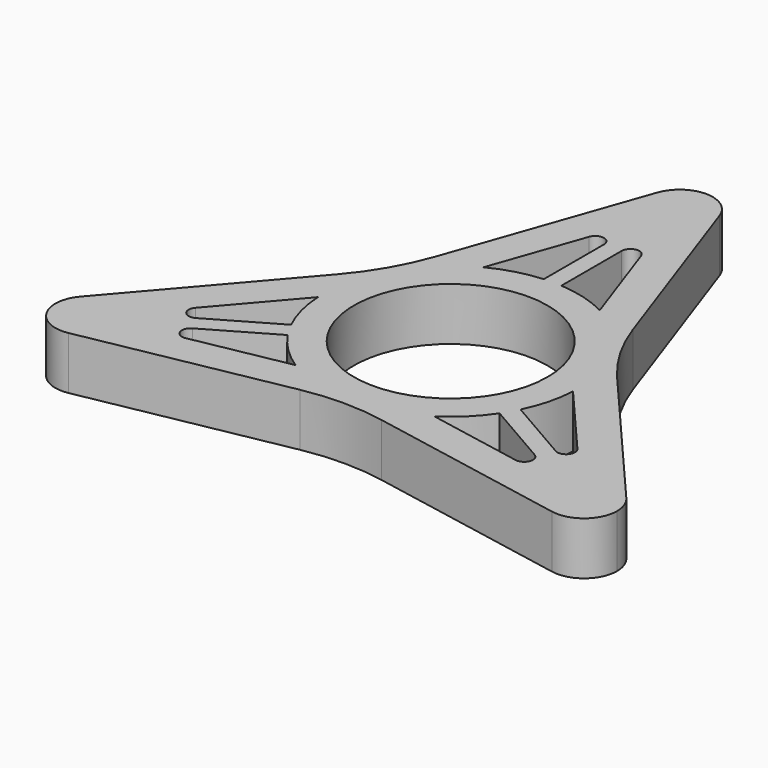
from build123d import *

# Parameters (mm, degrees)
F0_R     = 11
F1_DEPTH = 6


with BuildPart() as f1:
    # F0 (on Top) → F1 (new body)
    with BuildSketch(Plane.XY):
        with BuildLine():
            Line((11.2187429189, 11.8292181419), (3.5389187623, 33.7403846154))
            ThreePointArc((3.5389187623, 33.7403846154), (0, 36.25), (-3.5389187623, 33.7403846154))
            Line((-3.5389187623, 33.7403846154), (-11.2187429189, 11.8292181419))
            ThreePointArc((-11.2187429189, 11.8292181419), (-13.1608995727, 7.5984489111), (-15.8537748772, 3.8011072954))
            Line((-15.8537748772, 3.8011072954), (-30.9894895915, -13.8053987576))
            ThreePointArc((-30.9894895915, -13.8053987576), (-28.3703151015, -12.5067254343), (-25.6147048476, -13.4830653025))
            ThreePointArc((-25.6147048476, -13.4830653025), (-24.8982303588, -14.375), (-24.4840294966, -15.4414524572))
            ThreePointArc((-24.4840294966, -15.4414524572), (-24.4179418082, -15.8433278187), (-24.395825623, -16.25))
            ThreePointArc((-24.395825623, -16.25), (-25.2588111204, -18.643250355), (-27.4505708292, -19.9349858577))
            Line((-27.4505708292, -19.9349858577), (-4.6350319583, -15.6303254372))
            ThreePointArc((-4.6350319583, -15.6303254372), (0, -15.1968978222), (4.6350319583, -15.6303254372))
            Line((4.6350319583, -15.6303254372), (27.4505708292, -19.9349858577))
            ThreePointArc((27.4505708292, -19.9349858577), (25.016299495, -18.3160508741), (24.4840294966, -15.4414524572))
            ThreePointArc((24.4840294966, -15.4414524572), (24.8982303588, -14.375), (25.6147048476, -13.4830653025))
            ThreePointArc((25.6147048476, -13.4830653025), (28.3703151015, -12.5067254343), (30.9894895915, -13.8053987576))
            Line((30.9894895915, -13.8053987576), (15.8537748772, 3.8011072954))
            ThreePointArc((15.8537748772, 3.8011072954), (13.1608995727, 7.5984489111), (11.2187429189, 11.8292181419))
        make_face()
        with BuildLine():
            Line((-19.4313725784, -12.3734087272), (-12.0274698164, -8.0987634745))
            ThreePointArc((-12.0274698164, -8.0987634745), (-10.1599093098, -10.3453488494), (-7.8799155315, -12.171973185))
            Line((-7.8799155315, -12.171973185), (-18.7459713, -14.2220970264))
            ThreePointArc((-18.7459713, -14.2220970264), (-19.8690053401, -13.5870615238), (-19.4313725784, -12.3734087272))
        make_face(mode=Mode.SUBTRACT)
        with BuildLine():
            ThreePointArc((-20.4313725784, -10.6413579197), (-21.7012431124, -10.4135326105), (-21.68968297, -9.1234388512))
            Line((-21.68968297, -9.1234388512), (-14.4811957581, -0.7382204374))
            ThreePointArc((-14.4811957581, -0.7382204374), (-14.0392895695, -3.6260651377), (-13.0274698164, -6.366712667))
            Line((-13.0274698164, -6.366712667), (-20.4313725784, -10.6413579197))
        make_face(mode=Mode.SUBTRACT)
        with BuildLine():
            ThreePointArc((19.4313725784, -12.3734087272), (19.8690053401, -13.5870615238), (18.7459713, -14.2220970264))
            Line((18.7459713, -14.2220970264), (7.8799155315, -12.171973185))
            ThreePointArc((7.8799155315, -12.171973185), (10.1599093098, -10.3453488494), (12.0274698164, -8.0987634745))
            Line((12.0274698164, -8.0987634745), (19.4313725784, -12.3734087272))
        make_face(mode=Mode.SUBTRACT)
        Circle(F0_R, mode=Mode.SUBTRACT)
        with BuildLine():
            Line((14.4811957581, -0.7382204374), (21.68968297, -9.1234388512))
            ThreePointArc((21.68968297, -9.1234388512), (21.7012431124, -10.4135326105), (20.4313725784, -10.6413579197))
            Line((20.4313725784, -10.6413579197), (13.0274698164, -6.366712667))
            ThreePointArc((13.0274698164, -6.366712667), (14.0392895695, -3.6260651377), (14.4811957581, -0.7382204374))
        make_face(mode=Mode.SUBTRACT)
        with BuildLine():
            Line((-6.6012802267, 12.9101936225), (-2.9437116699, 23.3455358777))
            ThreePointArc((-2.9437116699, 23.3455358777), (-1.8322377723, 24.0005941343), (-1, 23.0147666469))
            Line((-1, 23.0147666469), (-1, 14.4654761415))
            ThreePointArc((-1, 14.4654761415), (-3.8793802597, 13.9714139872), (-6.6012802267, 12.9101936225))
        make_face(mode=Mode.SUBTRACT)
        with BuildLine():
            ThreePointArc((1, 23.0147666469), (1.8322377723, 24.0005941343), (2.9437116699, 23.3455358777))
            Line((2.9437116699, 23.3455358777), (6.6012802267, 12.9101936225))
            ThreePointArc((6.6012802267, 12.9101936225), (3.8793802597, 13.9714139872), (1, 14.4654761415))
            Line((1, 14.4654761415), (1, 23.0147666469))
        make_face(mode=Mode.SUBTRACT)
        with BuildLine():
            ThreePointArc((-25.6147048476, -13.4830653025), (-28.3703151015, -12.5067254343), (-30.9894895915, -13.8053987576))
            ThreePointArc((-30.9894895915, -13.8053987576), (-31.3934208872, -18.125), (-27.4505708292, -19.9349858577))
            ThreePointArc((-27.4505708292, -19.9349858577), (-25.2588111204, -18.643250355), (-24.395825623, -16.25))
            ThreePointArc((-24.395825623, -16.25), (-24.4179418082, -15.8433278187), (-24.4840294966, -15.4414524572))
            ThreePointArc((-24.4840294966, -15.4414524572), (-24.8982303588, -14.375), (-25.6147048476, -13.4830653025))
        make_face()
        with BuildLine():
            ThreePointArc((31.895825623, -16.25), (31.6619484793, -14.9463972771), (30.9894895915, -13.8053987576))
            ThreePointArc((30.9894895915, -13.8053987576), (28.3703151015, -12.5067254343), (25.6147048476, -13.4830653025))
            ThreePointArc((25.6147048476, -13.4830653025), (24.8982303588, -14.375), (24.4840294966, -15.4414524572))
            ThreePointArc((24.4840294966, -15.4414524572), (25.016299495, -18.3160508741), (27.4505708292, -19.9349858577))
            ThreePointArc((27.4505708292, -19.9349858577), (30.539075978, -19.1370145026), (31.895825623, -16.25))
        make_face()
    extrude(amount=F1_DEPTH)


solid = f1.part
